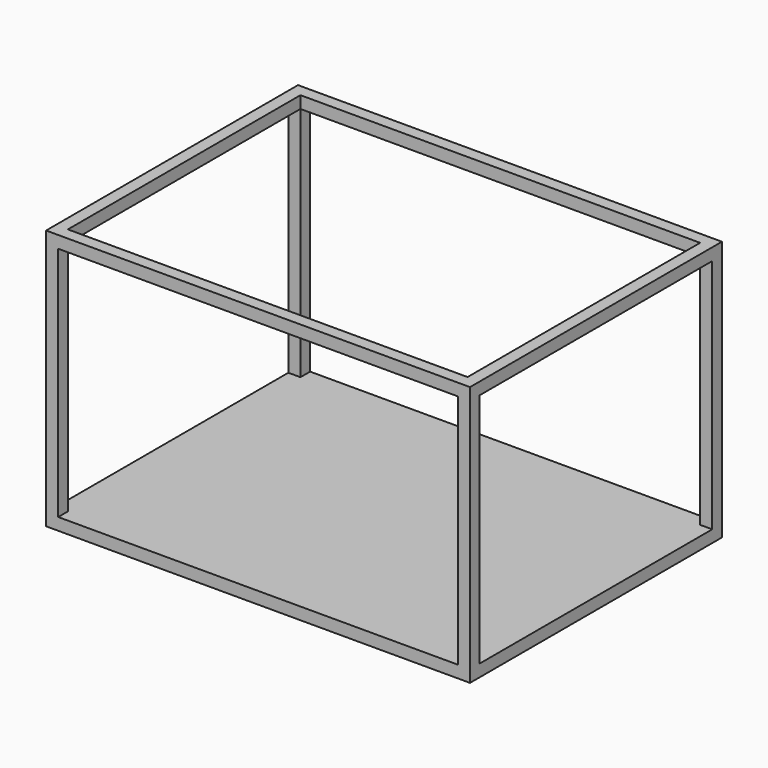
from build123d import *

# Parameters (mm, degrees)
F0_W      = 350
F0_H      = 215
F0_W_2    = 330
F0_H_2    = 195
F2_DEPTH  = 10
F1_W      = 260
F1_H      = 215
F1_W_2    = 240
F1_H_2    = 195
F3_DEPTH  = 10
F4_W      = 340
F4_H      = 240
F5_DEPTH  = 10
F8_W      = 350
F8_H      = 215
F8_W_2    = 330
F8_H_2    = 195
F10_DEPTH = 10
F9_W      = 260
F9_H      = 215
F9_W_2    = 240
F9_H_2    = 195
F11_DEPTH = 10


# Not quite as in the source:
# - a pattern or mirror of a feature is missing from the dataset's text; its kind, count and spacing are read off the source's solid


with BuildPart() as f2:
    # F0 (on Front) → F2 (new body, through all)
    with BuildSketch(Plane.XZ):
        with Locations((165, 97.5)):
            Rectangle(F0_W, F0_H)
        with Locations((165, 97.5)):
            Rectangle(F0_W_2, F0_H_2, mode=Mode.SUBTRACT)
    extrude(amount=-F2_DEPTH)


with BuildPart() as f2_copies_1:
    # F2_copies: instance of F2
    add(f2.part.mirror(Plane.ZX.offset(130)))


with BuildPart() as f2_1:
    add(f2.part)

    add(f2_copies_1.part)  # F3 merges F2_copies_1
    # F1 (on Right) → F3 (join, through all)
    with BuildSketch(Plane.YZ):
        with Locations((130, 97.5)):
            Rectangle(F1_W, F1_H)
        with Locations((130, 97.5)):
            Rectangle(F1_W_2, F1_H_2, mode=Mode.SUBTRACT)
    extrude(amount=-F3_DEPTH)

    # F4 (on face) → F5 (join, through all)
    with BuildSketch(Plane(origin=(0, 0, -10), x_dir=(1, 0, 0), z_dir=(0, 0, -1))):
        Polygon((340, -10), (340, 0), (-10.0000000001, 0), (-10.0000000001, -260), (340, -260), (340, -250), (0, -250), (0, -10), align=None)
        with Locations((170, -130)):
            Rectangle(F4_W, F4_H)
    extrude(amount=-F5_DEPTH)

    # F8 (on plane+point) → F10 (join, through all)
    with BuildSketch(Plane.XZ.offset(-260)):
        with Locations((165, 97.5)):
            Rectangle(F8_W, F8_H)
        with Locations((165, 97.5)):
            Rectangle(F8_W_2, F8_H_2, mode=Mode.SUBTRACT)
    extrude(amount=F10_DEPTH)

    # F9 (on plane+point) → F11 (join, through all)
    with BuildSketch(Plane.YZ.offset(340)):
        with Locations((130, 97.5)):
            Rectangle(F9_W, F9_H)
        with Locations((130, 97.5)):
            Rectangle(F9_W_2, F9_H_2, mode=Mode.SUBTRACT)
    extrude(amount=-F11_DEPTH)


solid = f2_1.part
